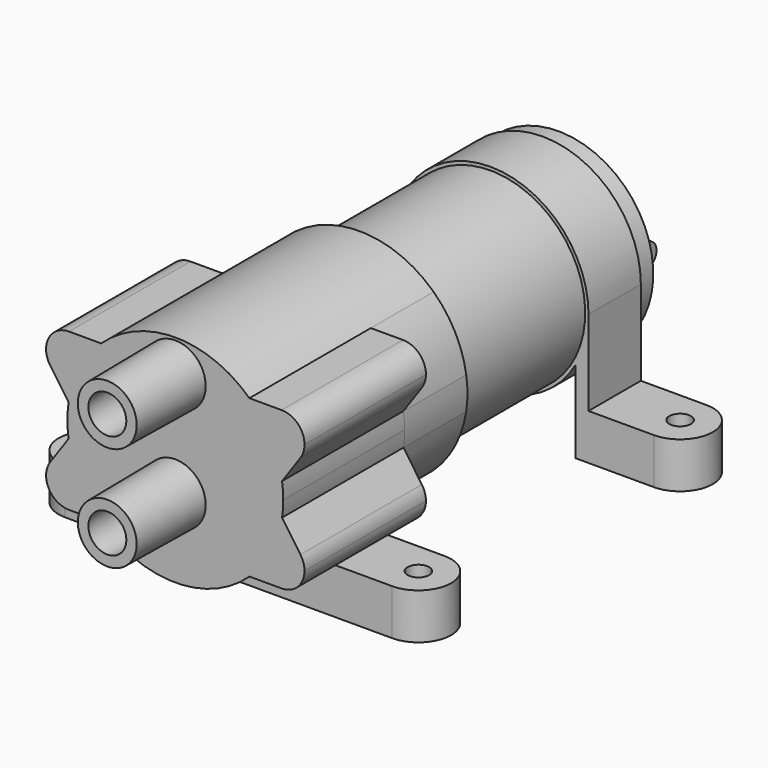
from build123d import *

# Parameters (mm, degrees)
F1_DEPTH  = 23.2
F6_DEPTH  = 12
F7_R      = 14.5
F8_DEPTH  = 38
F9_R      = 5
F10_DEPTH = 3
F9_W      = 0.8
F9_H      = 3.5
F11_DEPTH = 5
F12_R     = 1.74999
F14_R     = 1.65
F15_DEPTH = 7
F14_W     = 2
F14_H     = 10
F16_DEPTH = 20
F17_DEPTH = 7
F19_DEPTH = 10


# Not quite as in the source:
# - a fillet or chamfer is up to 0.001 mm smaller than in the source, because OpenCascade refuses the exact size


with BuildPart() as f1:
    # F0 (on Front) → F1 (new body)
    with BuildSketch(Plane.XZ):
        with BuildLine():
            ThreePointArc((16.315863747, -2.4581680554), (16.4539015408, -1.2325275198), (16.5, 0))
            ThreePointArc((16.5, 0), (16.4539015408, 1.2325275198), (16.315863747, 2.4581680554))
            ThreePointArc((16.315863747, 2.4581680554), (16.0653724653, 3.7621546421), (15.710839713, 5.0417770192))
            ThreePointArc((15.710839713, 5.0417770192), (13.1486562552, 6.8777586565), (13.1018809709, 10.0294922616))
            ThreePointArc((13.1018809709, 10.0294922616), (12.2529923089, 11.0505284706), (11.3247516529, 12))
            Line((11.3247516529, 12), (-11.3247516529, 12))
            ThreePointArc((-11.3247516529, 12), (-12.2529923089, 11.0505284706), (-13.1018809709, 10.0294922616))
            ThreePointArc((-13.1018809709, 10.0294922616), (-12.8391044723, 9.2847239636), (-12.75, 8.5))
            ThreePointArc((-12.75, 8.5), (-13.5913291851, 6.2237158574), (-15.710839713, 5.0417770192))
            ThreePointArc((-15.710839713, 5.0417770192), (-16.0653724653, 3.7621546421), (-16.315863747, 2.4581680554))
            ThreePointArc((-16.315863747, 2.4581680554), (-16.5, 0), (-16.315863747, -2.4581680554))
            ThreePointArc((-16.315863747, -2.4581680554), (-16.0653724653, -3.7621546421), (-15.710839713, -5.0417770192))
            ThreePointArc((-15.710839713, -5.0417770192), (-13.5913291851, -6.2237158574), (-12.75, -8.5))
            ThreePointArc((-12.75, -8.5), (-12.8391044723, -9.2847239636), (-13.1018809709, -10.0294922616))
            ThreePointArc((-13.1018809709, -10.0294922616), (-12.2529923089, -11.0505284706), (-11.3247516529, -12))
            Line((-11.3247516529, -12), (11.3247516529, -12))
            ThreePointArc((11.3247516529, -12), (12.2529923089, -11.0505284706), (13.1018809709, -10.0294922616))
            ThreePointArc((13.1018809709, -10.0294922616), (13.1486562552, -6.8777586566), (15.710839713, -5.0417770192))
            ThreePointArc((15.710839713, -5.0417770192), (16.0653724653, -3.7621546421), (16.315863747, -2.4581680554))
        make_face()
        with BuildLine():
            ThreePointArc((11.3247516529, 12), (12.2529923089, 11.0505284706), (13.1018809709, 10.0294922616))
            ThreePointArc((13.1018809709, 10.0294922616), (14.3930162784, 11.4667509936), (16.25, 12))
            Line((16.25, 12), (11.3247516529, 12))
        make_face()
        with BuildLine():
            ThreePointArc((-12.75, 8.5), (-12.8391044723, 9.2847239636), (-13.1018809709, 10.0294922616))
            ThreePointArc((-13.1018809709, 10.0294922616), (-14.6206205113, 7.6477091905), (-15.710839713, 5.0417770192))
            ThreePointArc((-15.710839713, 5.0417770192), (-13.5913291851, 6.2237158574), (-12.75, 8.5))
        make_face()
        with BuildLine():
            ThreePointArc((-15.710839713, 5.0417770192), (-14.6206205113, 7.6477091905), (-13.1018809709, 10.0294922616))
            ThreePointArc((-13.1018809709, 10.0294922616), (-14.3930162784, 11.4667509936), (-16.25, 12))
            ThreePointArc((-16.25, 12), (-19.3513437448, 10.1222413434), (-19.1249303104, 6.5038097008))
            ThreePointArc((-19.1249303104, 6.5038097008), (-17.627802704, 5.2826004741), (-15.710839713, 5.0417770192))
        make_face()
        with BuildLine():
            Line((-16.25, -12), (-11.3247516529, -12))
            ThreePointArc((-11.3247516529, -12), (-12.2529923089, -11.0505284706), (-13.1018809709, -10.0294922616))
            ThreePointArc((-13.1018809709, -10.0294922616), (-14.3930162784, -11.4667509936), (-16.25, -12))
        make_face()
        with BuildLine():
            Line((-11.3247516529, 12), (11.3247516529, 12))
            ThreePointArc((11.3247516529, 12), (0, 16.5), (-11.3247516529, 12))
        make_face()
        with BuildLine():
            Line((19.1249303104, -6.5038097008), (16.315863747, -2.4581680554))
            ThreePointArc((16.315863747, -2.4581680554), (16.0653724653, -3.7621546421), (15.710839713, -5.0417770192))
            ThreePointArc((15.710839713, -5.0417770192), (17.627802704, -5.2826004741), (19.1249303104, -6.5038097008))
        make_face()
        with BuildLine():
            ThreePointArc((13.1018809709, 10.0294922616), (14.6206205113, 7.6477091905), (15.710839713, 5.0417770192))
            ThreePointArc((15.710839713, 5.0417770192), (17.627802704, 5.2826004741), (19.1249303104, 6.5038097008))
            ThreePointArc((19.1249303104, 6.5038097008), (19.5900790474, 7.4541166619), (19.75, 8.5))
            ThreePointArc((19.75, 8.5), (18.7248737342, 10.9748737342), (16.25, 12))
            ThreePointArc((16.25, 12), (14.3930162784, 11.4667509936), (13.1018809709, 10.0294922616))
        make_face()
        with BuildLine():
            ThreePointArc((-16.25, -12), (-14.3930162784, -11.4667509936), (-13.1018809709, -10.0294922616))
            ThreePointArc((-13.1018809709, -10.0294922616), (-14.6206205113, -7.6477091905), (-15.710839713, -5.0417770192))
            ThreePointArc((-15.710839713, -5.0417770192), (-17.627802704, -5.2826004741), (-19.1249303104, -6.5038097008))
            ThreePointArc((-19.1249303104, -6.5038097008), (-19.3513437448, -10.1222413434), (-16.25, -12))
        make_face()
        with BuildLine():
            ThreePointArc((16.25, -12), (14.3930162784, -11.4667509936), (13.1018809709, -10.0294922616))
            ThreePointArc((13.1018809709, -10.0294922616), (12.2529923089, -11.0505284706), (11.3247516529, -12))
            Line((11.3247516529, -12), (16.25, -12))
        make_face()
        with BuildLine():
            ThreePointArc((19.1249303104, -6.5038097008), (17.627802704, -5.2826004741), (15.710839713, -5.0417770192))
            ThreePointArc((15.710839713, -5.0417770192), (14.6206205113, -7.6477091905), (13.1018809709, -10.0294922616))
            ThreePointArc((13.1018809709, -10.0294922616), (14.3930162784, -11.4667509936), (16.25, -12))
            ThreePointArc((16.25, -12), (18.7248737342, -10.9748737342), (19.75, -8.5))
            ThreePointArc((19.75, -8.5), (19.5900790474, -7.4541166619), (19.1249303104, -6.5038097008))
        make_face()
        with BuildLine():
            ThreePointArc((-13.1018809709, 10.0294922616), (-12.2529923089, 11.0505284706), (-11.3247516529, 12))
            Line((-11.3247516529, 12), (-16.25, 12))
            ThreePointArc((-16.25, 12), (-14.3930162784, 11.4667509936), (-13.1018809709, 10.0294922616))
        make_face()
        with BuildLine():
            ThreePointArc((15.710839713, 5.0417770192), (16.0653724653, 3.7621546421), (16.315863747, 2.4581680554))
            Line((16.315863747, 2.4581680554), (19.1249303104, 6.5038097008))
            ThreePointArc((19.1249303104, 6.5038097008), (17.627802704, 5.2826004741), (15.710839713, 5.0417770192))
        make_face()
        with BuildLine():
            ThreePointArc((13.1018809709, 10.0294922616), (13.1486562552, 6.8777586565), (15.710839713, 5.0417770192))
            ThreePointArc((15.710839713, 5.0417770192), (14.6206205113, 7.6477091905), (13.1018809709, 10.0294922616))
        make_face()
        with BuildLine():
            ThreePointArc((13.1018809709, -10.0294922616), (14.6206205113, -7.6477091905), (15.710839713, -5.0417770192))
            ThreePointArc((15.710839713, -5.0417770192), (13.1486562552, -6.8777586566), (13.1018809709, -10.0294922616))
        make_face()
        with BuildLine():
            ThreePointArc((-19.1249303104, -6.5038097008), (-17.627802704, -5.2826004741), (-15.710839713, -5.0417770192))
            ThreePointArc((-15.710839713, -5.0417770192), (-16.0653724653, -3.7621546421), (-16.315863747, -2.4581680554))
            Line((-16.315863747, -2.4581680554), (-19.1249303104, -6.5038097008))
        make_face()
        with BuildLine():
            ThreePointArc((-15.710839713, -5.0417770192), (-14.6206205113, -7.6477091905), (-13.1018809709, -10.0294922616))
            ThreePointArc((-13.1018809709, -10.0294922616), (-12.8391044723, -9.2847239636), (-12.75, -8.5))
            ThreePointArc((-12.75, -8.5), (-13.5913291851, -6.2237158574), (-15.710839713, -5.0417770192))
        make_face()
        with BuildLine():
            ThreePointArc((-16.315863747, 2.4581680554), (-16.0653724653, 3.7621546421), (-15.710839713, 5.0417770192))
            ThreePointArc((-15.710839713, 5.0417770192), (-17.627802704, 5.2826004741), (-19.1249303104, 6.5038097008))
            Line((-19.1249303104, 6.5038097008), (-16.315863747, 2.4581680554))
        make_face()
        with BuildLine():
            ThreePointArc((-11.3247516529, -12), (0, -16.5), (11.3247516529, -12))
            Line((11.3247516529, -12), (-11.3247516529, -12))
        make_face()
    extrude(amount=-F1_DEPTH)

    # F2 (on Right) → F3 (revolve)
    with BuildSketch(Plane.YZ):
        Polygon((0, 14.4998934947), (0, 16.1), (-13, 15.95), (-12.9815396904, 14.3501064982), align=None)
    revolve(axis=Axis((0, -6.5, 11.45), (0, -1, 0)))

    # F2 (on Right) → F4 (revolve)
    with BuildSketch(Plane.YZ):
        Polygon((0, -1.5001065053), (0, 0.1), (-13, -0.05), (-12.9815396904, -1.6498935018), align=None)
    revolve(axis=Axis((0, -6.5, -4.55), (0, -1, 0)))

    # F5 (on face) → F6 (join)
    with BuildSketch(Plane(origin=(0, 23.2, 0), x_dir=(-1, 0, 0), z_dir=(0, 1, 0))):
        with BuildLine():
            ThreePointArc((16.315863747, -2.4581680554), (16.4539015408, -1.2325275198), (16.5, 0))
            ThreePointArc((16.5, 0), (16.4539015408, 1.2325275198), (16.315863747, 2.4581680554))
            ThreePointArc((16.315863747, 2.4581680554), (14.6206205113, 7.6477091906), (11.3247516529, 12))
            ThreePointArc((11.3247516529, 12), (0, 16.5), (-11.3247516529, 12))
            ThreePointArc((-11.3247516529, 12), (-14.6206205113, 7.6477091906), (-16.315863747, 2.4581680554))
            ThreePointArc((-16.315863747, 2.4581680554), (-16.5, 0), (-16.315863747, -2.4581680554))
            ThreePointArc((-16.315863747, -2.4581680554), (-14.6206205113, -7.6477091905), (-11.3247516529, -12))
            ThreePointArc((-11.3247516529, -12), (0, -16.5), (11.3247516529, -12))
            ThreePointArc((11.3247516529, -12), (14.6206205113, -7.6477091906), (16.315863747, -2.4581680554))
        make_face()
    extrude(amount=F6_DEPTH)

    # F7 (on face) → F8 (join)
    with BuildSketch(Plane(origin=(0, 35.2, 0), x_dir=(-1, 0, 0), z_dir=(0, 1, 0))):
        Circle(F7_R)
    extrude(amount=F8_DEPTH)

    # F9 (on face) → F10 (join)
    with BuildSketch(Plane(origin=(0, 73.2, 0), x_dir=(-1, 0, 0), z_dir=(0, 1, 0))):
        Circle(F9_R)
    extrude(amount=F10_DEPTH)

    # F9 (on face) → F11 (join)
    with BuildSketch(Plane(origin=(0, 73.2, 0), x_dir=(-1, 0, 0), z_dir=(0, 1, 0))):
        with Locations((-10.6, 0)):
            Rectangle(F9_W, F9_H)
        with Locations((10.6, 0)):
            Rectangle(F9_W, F9_H)
    extrude(amount=F11_DEPTH)

    # F12 (radius 1.75 in the source; OpenCascade refuses exactly that, so slightly less here)
    f12_edges = [f1.edges().sort_by_distance(p)[0] for p in [
        (-10.6, 78.2, -1.75),
        (-10.6, 78.2, 1.75),
        (10.6, 78.2, -1.75),
        (10.6, 78.2, 1.75),
    ]]
    fillet(f12_edges, radius=F12_R)

    # F14 (on offset) → F15 (join)
    with BuildSketch(Plane.XY.offset(-20)):
        with BuildLine():
            ThreePointArc((-25, 20.2), (-30, 15.2), (-25, 10.2))
            Line((-25, 10.2), (25, 10.2))
            ThreePointArc((25, 10.2), (30, 15.2), (25, 20.2))
            Line((25, 20.2), (-25, 20.2))
        make_face()
        with Locations((-25, 15.2)):
            Circle(F14_R, mode=Mode.SUBTRACT)
        with Locations((25, 15.2)):
            Circle(F14_R, mode=Mode.SUBTRACT)
    extrude(amount=F15_DEPTH)

    # F14 (on offset) → F16 (join)
    with BuildSketch(Plane.XY.offset(-20)):
        with Locations((-14, 65.2)):
            Rectangle(F14_W, F14_H)
        with Locations((14, 65.2)):
            Rectangle(F14_W, F14_H)
    extrude(amount=F16_DEPTH)

    # F14 (on offset) → F17 (join)
    with BuildSketch(Plane.XY.offset(-20)):
        with BuildLine():
            ThreePointArc((-25, 70.2), (-30, 65.2), (-25, 60.2))
            Line((-25, 60.2), (-15, 60.2))
            Line((-15, 60.2), (-15, 70.2))
            Line((-15, 70.2), (-25, 70.2))
        make_face()
        with Locations((-25, 65.2)):
            Circle(F14_R, mode=Mode.SUBTRACT)
        with BuildLine():
            Line((15, 70.2), (15, 60.2))
            Line((15, 60.2), (25, 60.2))
            ThreePointArc((25, 60.2), (30, 65.2), (25, 70.2))
            Line((25, 70.2), (15, 70.2))
        make_face()
        with Locations((25, 65.2)):
            Circle(F14_R, mode=Mode.SUBTRACT)
    extrude(amount=F17_DEPTH)

    # F18 (on face) → F19 (join, through all)
    with BuildSketch(Plane(origin=(0, 70.2, 0), x_dir=(-1, 0, 0), z_dir=(0, 1, 0))):
        with BuildLine():
            Line((14.5, 0), (15, 0))
            ThreePointArc((15, 0), (-14.4913767462, 3.8729833462), (13, -7.4833147735))
            Line((13, -7.4833147735), (13, -6.4226162893))
            ThreePointArc((13, -6.4226162893), (14.1200212464, -3.2977264896), (14.5, 0))
        make_face()
    extrude(amount=-F19_DEPTH)


solid = f1.part
